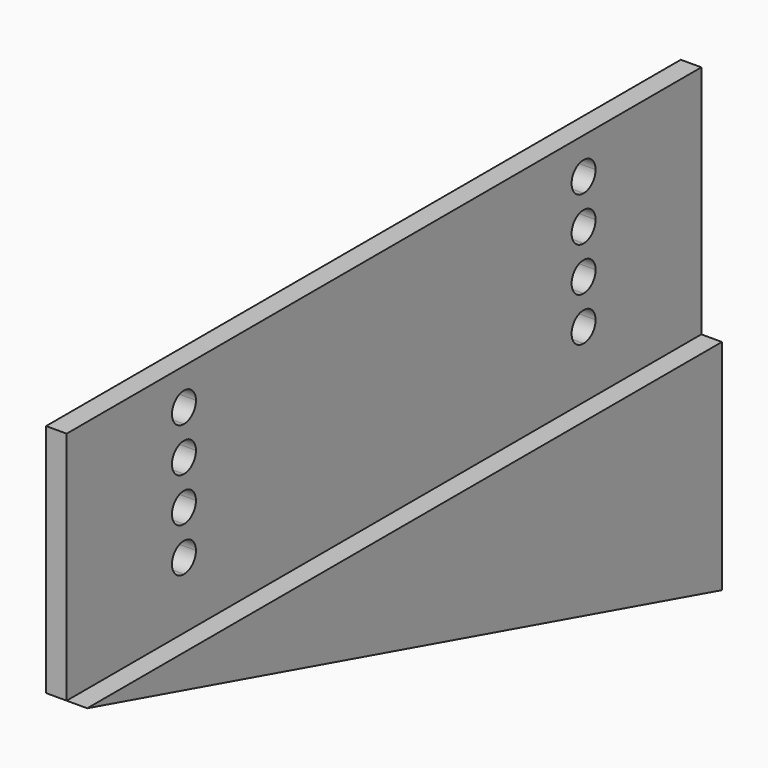
from build123d import *

# Parameters (mm, degrees)
F1_DEPTH = 7
F3_DEPTH = 14


# Not quite as in the source:
# - a feature names something its author has since deleted; it is built from what else it names


with BuildPart() as f1:
    # F0 (on Right) → F1 (new body)
    with BuildSketch(Plane.YZ):
        Polygon((-102.4108821703, 80), (-152.4108821703, 80), (-152.4108821703, 0), (117.5891178297, 0), (117.5891178297, 80), (67.5891178297, 80), align=None)
        with BuildLine():
            ThreePointArc((-102.4608821703, 27.6177177185), (-98.8930703505, 26.1711353257), (-97.4108821703, 22.6179677248))
            ThreePointArc((-97.4108821703, 22.6179677248), (-98.8930703505, 19.0648001239), (-102.4608821703, 17.6182177311))
            ThreePointArc((-102.4608821703, 17.6182177311), (-102.5108821703, 17.6179677248), (-102.5608821703, 17.6182177311))
            ThreePointArc((-102.5608821703, 17.6182177311), (-107.6108821703, 22.6179677248), (-102.5608821703, 27.6177177185))
            ThreePointArc((-102.5608821703, 27.6177177185), (-102.5108821703, 27.6179677248), (-102.4608821703, 27.6177177185))
        make_face(mode=Mode.SUBTRACT)
        with BuildLine():
            ThreePointArc((-102.4608821703, 42.6177177185), (-98.8930703505, 41.1711353257), (-97.4108821703, 37.6179677248))
            ThreePointArc((-97.4108821703, 37.6179677248), (-98.8930703505, 34.0648001239), (-102.4608821703, 32.6182177311))
            ThreePointArc((-102.4608821703, 32.6182177311), (-102.5108821703, 32.6179677248), (-102.5608821703, 32.6182177311))
            ThreePointArc((-102.5608821703, 32.6182177311), (-107.6108821703, 37.6179677248), (-102.5608821703, 42.6177177185))
            ThreePointArc((-102.5608821703, 42.6177177185), (-102.5108821703, 42.6179677248), (-102.4608821703, 42.6177177185))
        make_face(mode=Mode.SUBTRACT)
        with BuildLine():
            ThreePointArc((-102.4608821703, 57.6177177185), (-98.8930703505, 56.1711353257), (-97.4108821703, 52.6179677248))
            ThreePointArc((-97.4108821703, 52.6179677248), (-98.8930703505, 49.0648001239), (-102.4608821703, 47.6182177311))
            ThreePointArc((-102.4608821703, 47.6182177311), (-102.5108821703, 47.6179677248), (-102.5608821703, 47.6182177311))
            ThreePointArc((-102.5608821703, 47.6182177311), (-107.6108821703, 52.6179677248), (-102.5608821703, 57.6177177185))
            ThreePointArc((-102.5608821703, 57.6177177185), (-102.5108821703, 57.6179677248), (-102.4608821703, 57.6177177185))
        make_face(mode=Mode.SUBTRACT)
        with BuildLine():
            ThreePointArc((-102.4608821703, 72.6177177185), (-98.8930703505, 71.1711353257), (-97.4108821703, 67.6179677248))
            ThreePointArc((-97.4108821703, 67.6179677248), (-98.8930703505, 64.0648001239), (-102.4608821703, 62.6182177311))
            ThreePointArc((-102.4608821703, 62.6182177311), (-102.5108821703, 62.6179677248), (-102.5608821703, 62.6182177311))
            ThreePointArc((-102.5608821703, 62.6182177311), (-107.6108821703, 67.6179677248), (-102.5608821703, 72.6177177185))
            ThreePointArc((-102.5608821703, 72.6177177185), (-102.5108821703, 72.6179677248), (-102.4608821703, 72.6177177185))
        make_face(mode=Mode.SUBTRACT)
        with BuildLine():
            ThreePointArc((67.5391178297, 27.6177177185), (71.1069296495, 26.1711353257), (72.5891178297, 22.6179677248))
            ThreePointArc((72.5891178297, 22.6179677248), (71.1069296495, 19.0648001239), (67.5391178297, 17.6182177311))
            ThreePointArc((67.5391178297, 17.6182177311), (67.4891178297, 17.6179677248), (67.4391178297, 17.6182177311))
            ThreePointArc((67.4391178297, 17.6182177311), (62.3891178297, 22.6179677248), (67.4391178297, 27.6177177185))
            ThreePointArc((67.4391178297, 27.6177177185), (67.4891178297, 27.6179677248), (67.5391178297, 27.6177177185))
        make_face(mode=Mode.SUBTRACT)
        with BuildLine():
            ThreePointArc((67.5391178297, 42.6177177185), (71.1069296495, 41.1711353257), (72.5891178297, 37.6179677248))
            ThreePointArc((72.5891178297, 37.6179677248), (71.1069296495, 34.0648001239), (67.5391178297, 32.6182177311))
            ThreePointArc((67.5391178297, 32.6182177311), (67.4891178297, 32.6179677248), (67.4391178297, 32.6182177311))
            ThreePointArc((67.4391178297, 32.6182177311), (62.3891178297, 37.6179677248), (67.4391178297, 42.6177177185))
            ThreePointArc((67.4391178297, 42.6177177185), (67.4891178297, 42.6179677248), (67.5391178297, 42.6177177185))
        make_face(mode=Mode.SUBTRACT)
        with BuildLine():
            ThreePointArc((67.5391178297, 57.6177177185), (71.1069296495, 56.1711353257), (72.5891178297, 52.6179677248))
            ThreePointArc((72.5891178297, 52.6179677248), (71.1069296495, 49.0648001239), (67.5391178297, 47.6182177311))
            ThreePointArc((67.5391178297, 47.6182177311), (67.4891178297, 47.6179677248), (67.4391178297, 47.6182177311))
            ThreePointArc((67.4391178297, 47.6182177311), (62.3891178297, 52.6179677248), (67.4391178297, 57.6177177185))
            ThreePointArc((67.4391178297, 57.6177177185), (67.4891178297, 57.6179677248), (67.5391178297, 57.6177177185))
        make_face(mode=Mode.SUBTRACT)
        with BuildLine():
            ThreePointArc((67.5391178297, 72.6177177185), (71.1069296495, 71.1711353257), (72.5891178297, 67.6179677248))
            ThreePointArc((72.5891178297, 67.6179677248), (71.1069296495, 64.0648001239), (67.5391178297, 62.6182177311))
            ThreePointArc((67.5391178297, 62.6182177311), (67.4891178297, 62.6179677248), (67.4391178297, 62.6182177311))
            ThreePointArc((67.4391178297, 62.6182177311), (62.3891178297, 67.6179677248), (67.4391178297, 72.6177177185))
            ThreePointArc((67.4391178297, 72.6177177185), (67.4891178297, 72.6179677248), (67.5391178297, 72.6177177185))
        make_face(mode=Mode.SUBTRACT)
        Polygon((117.5891178297, 0), (-152.4108821703, 0), (117.5891178297, -74.3703905304), align=None)
    extrude(amount=F1_DEPTH)

    # F2 (on face) → F3 (join)
    with BuildSketch(Plane(origin=(0, 0, 0), x_dir=(0, -1, 0), z_dir=(-1, 0, 0))):
        Polygon((-117.5891178297, -74.3703905304), (152.4108821703, 0), (-117.5891178297, 0), align=None)
    extrude(amount=-F3_DEPTH)


solid = f1.part
